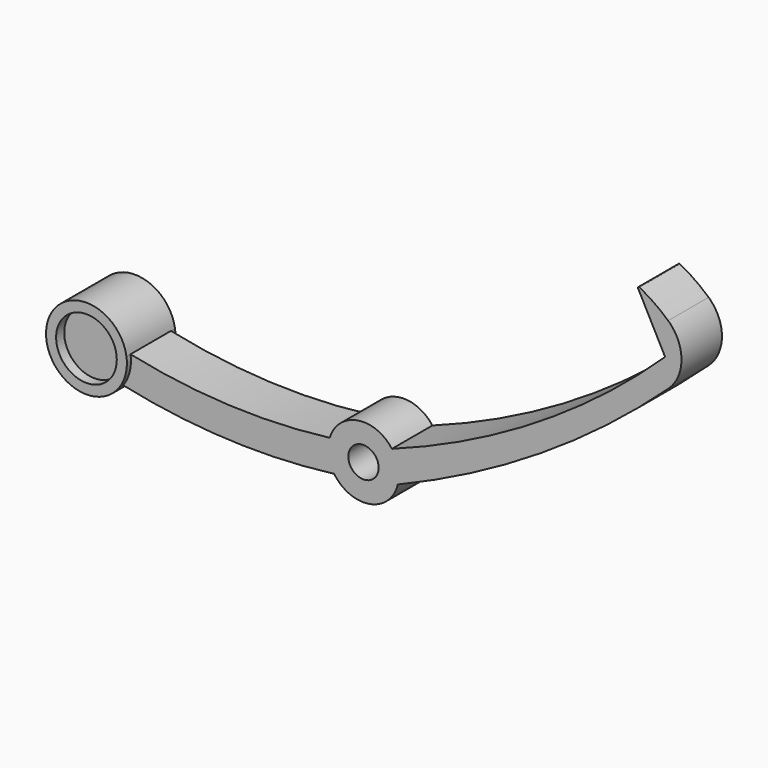
from build123d import *

# Parameters (mm, degrees)
F0_R     = 1.5
F1_DEPTH = 2.5
F0_R_2   = 3
F2_DEPTH = 3
F3_DEPTH = 2
F4_R     = 4
F5_R     = 0.1


# Not quite as in the source:
# - a feature names something its author has since deleted; it is built from what else it names


with BuildPart() as f1:
    # F0 (on Front) → F1 (new body, symmetric)
    with BuildSketch(Plane.XZ):
        with BuildLine():
            ThreePointArc((-26.557532, -71.276034), (-16.16683, -72.628107), (-5.697339, -72.198498))
            ThreePointArc((-5.697339, -72.198498), (-2.181593, -73.689218), (0.604666, -71.077807))
            ThreePointArc((0.604666, -71.077807), (16.299458, -62.740057), (30.034164, -51.461652))
            ThreePointArc((30.034164, -51.461652), (27.535845, -48.296422), (24.222658, -45.99793))
            Line((24.222658, -45.99793), (27.041809, -51.380895))
            ThreePointArc((27.041809, -51.380895), (14.399768, -61.170328), (0.02157, -68.164727))
            ThreePointArc((0.02157, -68.164727), (-3.377934, -66.79227), (-6.137191, -69.20614))
            ThreePointArc((-6.137191, -69.20614), (-16.024246, -69.607733), (-25.837738, -68.338673))
            ThreePointArc((-25.837738, -68.338673), (-25.80524, -68.631526), (-25.794387, -68.925977))
            ThreePointArc((-25.794387, -68.925977), (-25.989954, -70.161408), (-26.557532, -71.276034))
        make_face()
        with Locations((-2.794387, -70.243281)):
            Circle(F0_R, mode=Mode.SUBTRACT)
    extrude(amount=F1_DEPTH, both=True)

    # F0 (on Front) → F2 (join, symmetric)
    with BuildSketch(Plane.XZ):
        with BuildLine():
            ThreePointArc((-25.837738, -68.338673), (-33.679442, -67.973952), (-26.557532, -71.276034))
            ThreePointArc((-26.557532, -71.276034), (-25.989954, -70.161408), (-25.794387, -68.925977))
            ThreePointArc((-25.794387, -68.925977), (-25.80524, -68.631526), (-25.837738, -68.338673))
        make_face()
        with Locations((-29.794387, -68.925977)):
            Circle(F0_R_2, mode=Mode.SUBTRACT)
    extrude(amount=F2_DEPTH, both=True)

    # F0 (on Front) → F3 (join, symmetric)
    with BuildSketch(Plane.XZ):
        with Locations((-29.794387, -68.925977)):
            Circle(F0_R_2)
    extrude(amount=F3_DEPTH, both=True)

    # F4
    f4_edges = [f1.edges().sort_by_distance(p)[0] for p in [
        (30.034164, 0, -51.461652),
    ]]
    fillet(f4_edges, radius=F4_R)

    # F5
    f5_edges = [f1.edges().sort_by_distance(p)[0] for p in [
        (24.222658, 0, -45.99793),
    ]]
    fillet(f5_edges, radius=F5_R)


solid = f1.part
